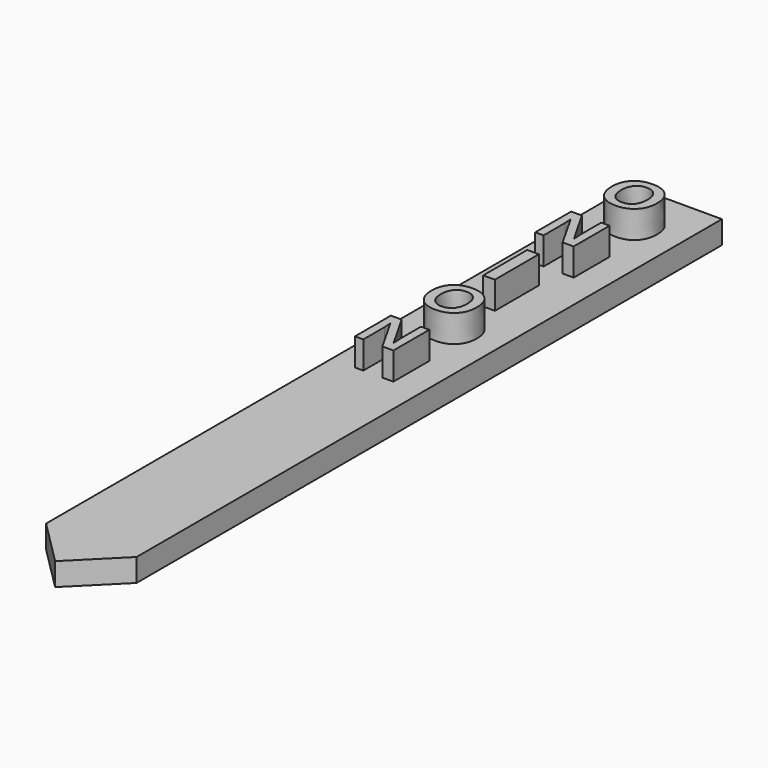
from build123d import *

# Parameters (mm, degrees)
F1_DEPTH       = 2.5
F2_TEXT_SIZE   = 7.1414709878
F2_TEXT_SIZE_2 = 8.4274603675
F3_DEPTH       = 3


# Not quite as in the source:
# - Text() gives the source's letters only with a copy of the font that has no kerning and outlines rounded to 1/6400 em; it was checked with that copy


with BuildPart() as f1:
    # F0 (on Top) → F1 (new body)
    with BuildSketch(Plane.XY):
        Polygon((-4.9497474683, 4.9497474683), (0, 0), (4.9497474683, 4.9497474683), (4.9497474683, 84.9497474683), (-4.9497474683, 84.9497474683), align=None)
    extrude(amount=F1_DEPTH)

    # F2 (on face) → F3 (join)
    with BuildSketch(Plane.XY.offset(2.5)):
        with Locations((-2.8579389353, 76.8078883571)):
            Text('O', F2_TEXT_SIZE, font='Arimo', font_style=FontStyle.BOLD, text_align=(TextAlign.LEFT, TextAlign.BOTTOM))
        with Locations((-2.8579389353, 68.5951967212)):
            Text('N', F2_TEXT_SIZE, font='Arimo', font_style=FontStyle.BOLD, text_align=(TextAlign.LEFT, TextAlign.BOTTOM))
        with Locations((-2.8579389353, 52.1698134493)):
            Text('O', F2_TEXT_SIZE, font='Arimo', font_style=FontStyle.BOLD, text_align=(TextAlign.LEFT, TextAlign.BOTTOM))
        with Locations((-2.8579389353, 43.9571218133)):
            Text('N', F2_TEXT_SIZE, font='Arimo', font_style=FontStyle.BOLD, text_align=(TextAlign.LEFT, TextAlign.BOTTOM))
        with Locations((-1.6298454786, 59.6010945737)):
            Text('I', F2_TEXT_SIZE_2, font='Open Sans', font_style=FontStyle.BOLD, text_align=(TextAlign.LEFT, TextAlign.BOTTOM))
    extrude(amount=F3_DEPTH)


solid = f1.part
